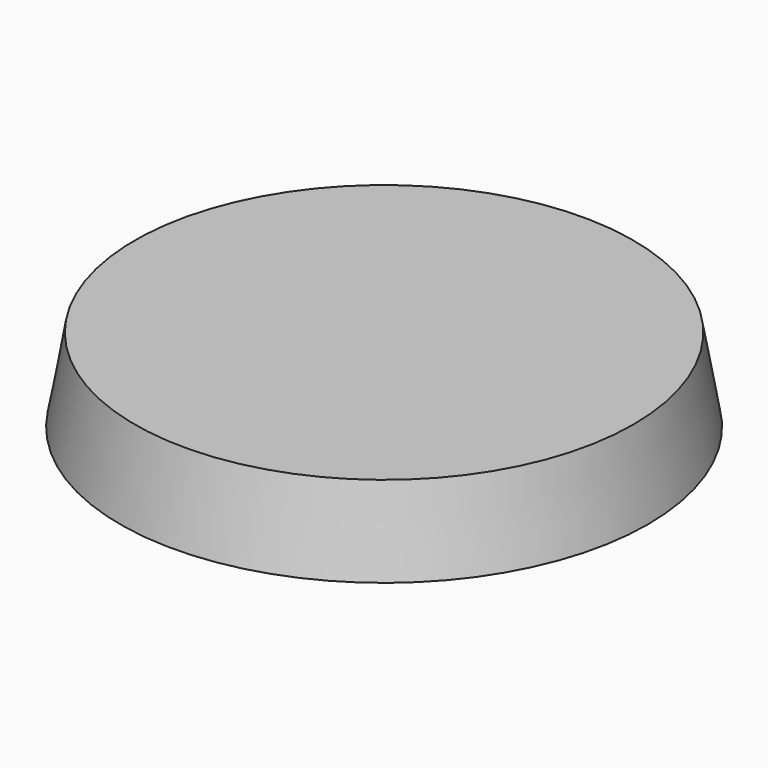
from build123d import *

# Parameters (mm, degrees)
F0_R           = 30
F1_DEPTH       = 10
F1_TAPER       = -10
F2_TEXT_SIZE   = 20.1131363922
F2_TEXT_SIZE_2 = 19.3374718453
F3_DEPTH       = 1


# Not quite as in the source:
# - Text() gives the source's letters only with a copy of the font that has no kerning and outlines rounded to 1/6400 em; it was checked with that copy


with BuildPart() as f1:
    # F0 (on Top) → F1 (new body)
    with BuildSketch(Plane.XY):
        Circle(F0_R)
    extrude(amount=-F1_DEPTH, taper=F1_TAPER)

    # F2 (on face) → F3 (cut)
    with BuildSketch(Plane(origin=(0, 0, -10), x_dir=(1, 0, 0), z_dir=(0, 0, -1))):
        with Locations((-15, 5.5185417976)):
            Text('LGJ', F2_TEXT_SIZE, font='Open Sans', font_style=FontStyle.ITALIC, text_align=(TextAlign.LEFT, TextAlign.BOTTOM))
        with Locations((-27, -10.9229797286)):
            Text('Ihrene', F2_TEXT_SIZE_2, font='Open Sans', font_style=FontStyle.ITALIC, text_align=(TextAlign.LEFT, TextAlign.BOTTOM))
    extrude(amount=-F3_DEPTH, mode=Mode.SUBTRACT)


solid = f1.part
